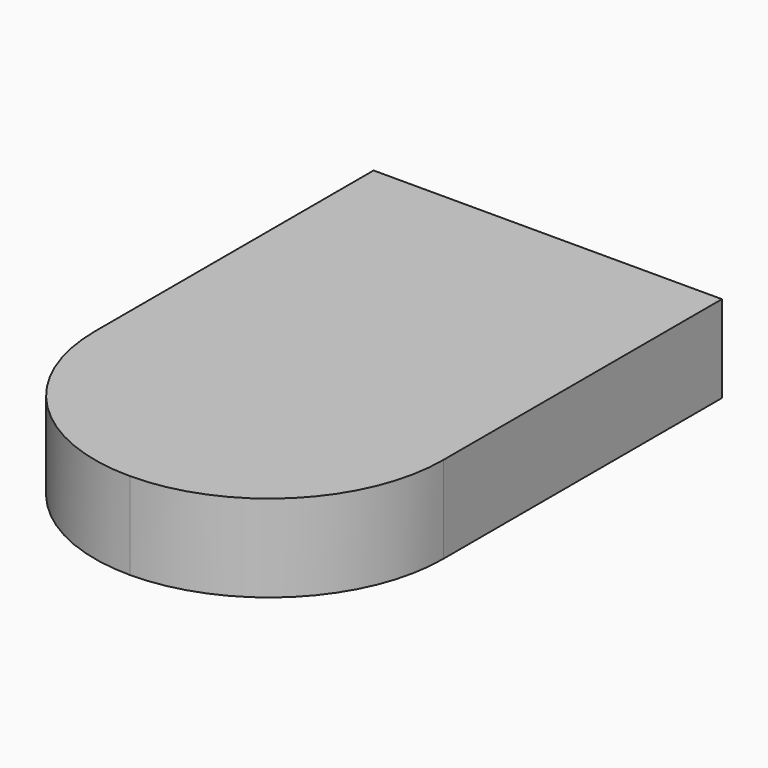
from build123d import *

# Parameters (mm, degrees)
F0_W     = 12.7
F0_H     = 19.05
F1_DEPTH = 3.175
F2_R     = 6.34999


# Not quite as in the source:
# - a fillet or chamfer is up to 0.001 mm smaller than in the source, because OpenCascade refuses the exact size


with BuildPart() as f1:
    # F0 (on Top) → F1 (new body)
    with BuildSketch(Plane.XY):
        with Locations((6.35, 9.525)):
            Rectangle(F0_W, F0_H)
    extrude(amount=F1_DEPTH)

    # F2 (radius 6.35 in the source; OpenCascade refuses exactly that, so slightly less here)
    f2_edges = [f1.edges().sort_by_distance(p)[0] for p in [
        (0, 0, 1.5875),
        (12.7, 0, 1.5875),
    ]]
    fillet(f2_edges, radius=F2_R)


solid = f1.part
